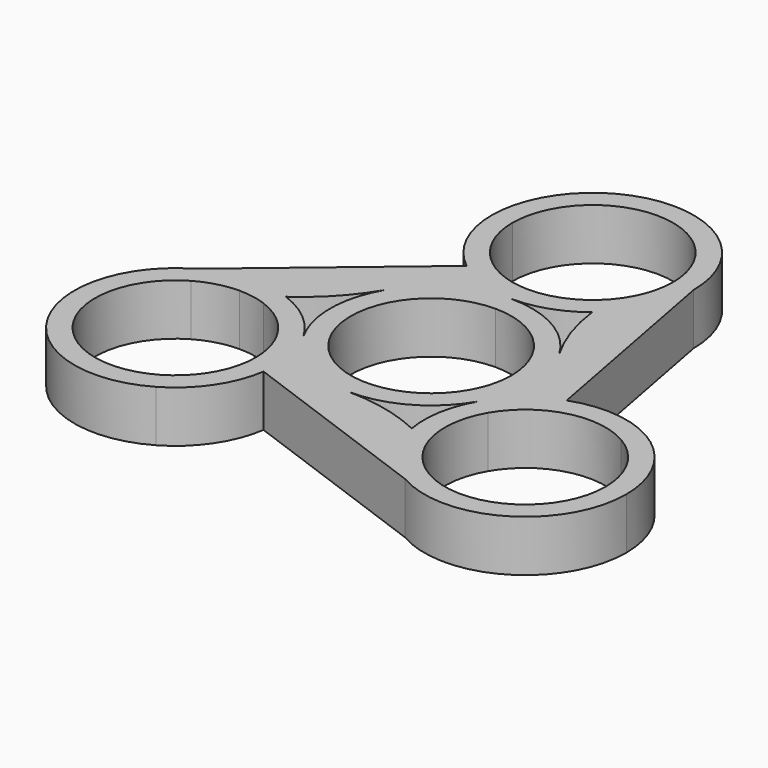
from build123d import *

# Parameters (mm, degrees)
F1_DEPTH = 7.112


# Not quite as in the source:
# - ends of sketch curves that miss each other by under 0.0002 mm in the source are joined
# - a feature names something its author has since deleted; it is built from what else it names


with BuildPart() as f1:
    # F0 (on Top) → F1 (new body)
    with BuildSketch(Plane.XY):
        with BuildLine():
            ThreePointArc((0, 11.1125), (7.8577241059, 7.8577241059), (11.1125, 0))
            ThreePointArc((11.1125, 0), (10.7338507446, -2.8761266387), (9.6237072996, -5.55625))
            Line((9.6237072996, -5.55625), (12.0983748909, -6.985))
            ThreePointArc((12.0983748909, -6.985), (13.4939838315, -3.6157019175), (13.97, 0))
            ThreePointArc((13.97, 0), (13.4755323786, 3.6838739276), (12.0271328398, 7.1069666985))
            ThreePointArc((12.0271328398, 7.1069666985), (6.9237480813, 12.133532565), (-1.95e-08, 13.97))
            Line((-1.95e-08, 13.97), (0, 11.1125))
        make_face()
        with BuildLine():
            ThreePointArc((-9.6237072996, -5.55625), (-9.6237072996, 5.55625), (0, 11.1125))
            Line((0, 11.1125), (0, 13.97))
            ThreePointArc((-1.95e-08, 13.97), (-6.9237478038, 12.1335327234), (-12.0271324949, 7.1069672823))
            ThreePointArc((-12.0271324949, 7.1069672823), (-13.9698214779, 0.0706248839), (-12.0983748909, -6.985))
            Line((-12.0983748909, -6.985), (-9.6237072996, -5.55625))
        make_face()
        with BuildLine():
            Line((12.0983748909, -6.985), (9.6237072996, -5.55625))
            ThreePointArc((9.6237072996, -5.55625), (0, -11.1125), (-9.6237072996, -5.55625))
            Line((-9.6237072996, -5.55625), (-12.0983748909, -6.985))
            ThreePointArc((-12.0983748909, -6.985), (-7.0460734842, -12.0629079602), (-0.1412475033, -13.969285921))
            ThreePointArc((-0.1412475033, -13.969285921), (6.9237481232, -12.1335325411), (12.0983748909, -6.985))
        make_face()
        with BuildLine():
            ThreePointArc((-8.6769039474, 16.9913819188), (-4.593947408, 14.7469507993), (-1.95e-08, 13.97))
            Line((0, 13.97), (0, 16.8275))
            ThreePointArc((0, 16.8275), (-3.65427634, 17.4455290423), (-6.9020826854, 19.2308719809))
            Line((-6.9020826854, 19.2308719809), (-8.6769039474, 16.9913819188))
        make_face()
        with BuildLine():
            ThreePointArc((-12.0271324949, 7.1069672823), (-6.9237478038, 12.1335327234), (-1.95e-08, 13.97))
            ThreePointArc((-1.95e-08, 13.97), (-4.593947408, 14.7469507993), (-8.6769039474, 16.9913819188))
            ThreePointArc((-8.6769039474, 16.9913819188), (-9.8388621787, 11.8752452293), (-12.0271324949, 7.1069672823))
        make_face()
        with BuildLine():
            Line((0, 16.8275), (0, 13.97))
            ThreePointArc((-1.95e-08, 13.97), (4.5939473896, 14.7469507929), (8.6769039474, 16.9913819188))
            ThreePointArc((8.6769039474, 16.9913819188), (12.5773059147, 21.8595168015), (13.97, 27.94))
            Line((13.97, 27.94), (11.1125, 27.94))
            ThreePointArc((11.1125, 27.94), (7.8577241059, 20.0822758941), (0, 16.8275))
        make_face()
        with BuildLine():
            ThreePointArc((19.4187283795, -0.8424940876), (15.2170069875, -3.2683590347), (12.0983750385, -6.9849997443))
            Line((12.0983750385, -6.9849997443), (14.5730424822, -8.41375))
            ThreePointArc((14.5730424822, -8.41375), (21.320623143, -3.2361492554), (29.7529997817, -4.3462927004))
            Line((29.7529997817, -4.3462927004), (31.1817497817, -1.8716251091))
            ThreePointArc((31.1817497817, -1.8716251091), (25.4143155079, -0.0531600677), (19.4187283795, -0.8424940876))
        make_face()
        with BuildLine():
            ThreePointArc((13.97, 0), (13.4939838315, -3.6157019175), (12.0983750385, -6.9849997443))
            ThreePointArc((12.0983750385, -6.9849997443), (15.2170069875, -3.2683590347), (19.4187283795, -0.8424940876))
            ThreePointArc((19.4187283795, -0.8424940876), (15.2933094518, 2.7327644521), (12.0271328398, 7.1069666985))
            ThreePointArc((12.0271328398, 7.1069666985), (13.4755323786, 3.6838739276), (13.97, 0))
        make_face()
        with BuildLine():
            Line((14.5730424822, -8.41375), (12.0983748909, -6.985))
            ThreePointArc((12.0983748909, -6.985), (10.4389854978, -11.5441348126), (10.4389854722, -16.395865042))
            ThreePointArc((10.4389854722, -16.395865042), (12.753195723, -21.9828628158), (17.2117497817, -26.0683748909))
            Line((17.2117497817, -26.0683748909), (18.6404997817, -23.5937072996))
            ThreePointArc((18.6404997817, -23.5937072996), (13.4628990371, -16.8461266387), (14.5730424822, -8.41375))
        make_face()
        with BuildLine():
            ThreePointArc((-10.2267497817, -13.97), (-10.7027659885, -10.3542979399), (-12.0983748909, -6.985))
            Line((-12.0983748909, -6.985), (-14.5730424822, -8.41375))
            ThreePointArc((-14.5730424822, -8.41375), (-13.4628990371, -11.0938733613), (-13.0842497817, -13.97))
            ThreePointArc((-13.0842497817, -13.97), (-14.5730424822, -19.52625), (-18.6404997817, -23.5937072996))
            Line((-18.6404997817, -23.5937072996), (-17.2117497817, -26.0683748909))
            ThreePointArc((-17.2117497817, -26.0683748909), (-12.6422439072, -21.8220248341), (-10.3765164134, -16.010110204))
            ThreePointArc((-10.3765164134, -16.010110204), (-10.2642417492, -14.9928000402), (-10.2267497817, -13.97))
        make_face()
        with BuildLine():
            ThreePointArc((-0.1412475033, -13.969285921), (-7.0460734842, -12.0629079602), (-12.0983748909, -6.985))
            ThreePointArc((-12.0983748909, -6.985), (-10.7027659885, -10.3542979399), (-10.2267497817, -13.97))
            ThreePointArc((-10.2267497817, -13.97), (-10.2642417492, -14.9928000402), (-10.3765164134, -16.010110204))
            ThreePointArc((-10.3765164134, -16.010110204), (-5.36483273, -14.4583271608), (-0.1412475033, -13.969285921))
        make_face()
        with BuildLine():
            Line((-14.5730424822, -8.41375), (-12.0983748909, -6.985))
            ThreePointArc((-12.0983748909, -6.985), (-15.2170068744, -3.2683591296), (-19.4187283795, -0.8424940876))
            Line((-19.4187283795, -0.8424940876), (-20.396050939, -3.5276657515))
            ThreePointArc((-20.396050939, -3.5276657515), (-17.0537724691, -5.4573311258), (-14.5730424822, -8.41375))
        make_face()
        with BuildLine():
            ThreePointArc((8.6769039474, 16.9913819188), (9.8388622875, 11.8752449082), (12.0271328398, 7.1069666985))
            ThreePointArc((12.0271328398, 7.1069666985), (15.2933094518, 2.7327644521), (19.4187283795, -0.8424940876))
            Line((19.4187283795, -0.8424940876), (13.97, 27.94))
            ThreePointArc((13.97, 27.94), (12.5773059147, 21.8595168015), (8.6769039474, 16.9913819188))
        make_face()
        with BuildLine():
            ThreePointArc((-19.4187283795, -0.8424940876), (-15.293309221, 2.7327647003), (-12.0271324949, 7.1069672823))
            ThreePointArc((-12.0271324949, 7.1069672823), (-9.8388621787, 11.8752452293), (-8.6769039474, 16.9913819188))
            Line((-8.6769039474, 16.9913819188), (-31.1817497817, -1.8716251091))
            ThreePointArc((-31.1817497817, -1.8716251091), (-27.8124518418, -0.4760162067), (-24.1967497817, 0))
            ThreePointArc((-24.1967497817, 0), (-21.7708847397, -0.2122356904), (-19.4187283795, -0.8424940876))
        make_face()
        with BuildLine():
            ThreePointArc((-13.97, 27.94), (-12.5773059147, 21.8595168015), (-8.6769039474, 16.9913819188))
            Line((-8.6769039474, 16.9913819188), (-6.9020826854, 19.2308719809))
            ThreePointArc((-6.9020826854, 19.2308719809), (-10.0046751594, 23.1032520012), (-11.1125, 27.94))
            Line((-11.1125, 27.94), (-13.97, 27.94))
        make_face()
        with BuildLine():
            ThreePointArc((10.4389854722, -16.395865042), (5.2800111814, -14.6107766948), (-0.1412475033, -13.969285921))
            ThreePointArc((-0.1412475033, -13.969285921), (-5.36483273, -14.4583271608), (-10.3765164134, -16.010110204))
            Line((-10.3765164134, -16.010110204), (17.2117497817, -26.0683748909))
            ThreePointArc((17.2117497817, -26.0683748909), (12.753195723, -21.9828628158), (10.4389854722, -16.395865042))
        make_face()
        with BuildLine():
            Line((-20.396050939, -3.5276657515), (-19.4187283795, -0.8424940876))
            ThreePointArc((-19.4187283795, -0.8424940876), (-21.7708847397, -0.2122356904), (-24.1967497817, 0))
            Line((-24.1967497817, 0), (-24.1967497817, -2.8575))
            ThreePointArc((-24.1967497817, -2.8575), (-22.2670844074, -3.0263238447), (-20.396050939, -3.5276657515))
        make_face()
        with BuildLine():
            ThreePointArc((-11.1125, 27.94), (0, 39.0525), (11.1125, 27.94))
            Line((11.1125, 27.94), (13.97, 27.94))
            ThreePointArc((13.97, 27.94), (0, 41.91), (-13.97, 27.94))
            Line((-13.97, 27.94), (-11.1125, 27.94))
        make_face()
        with BuildLine():
            Line((-29.7529997817, -4.3462927004), (-31.1817497817, -1.8716251091))
            ThreePointArc((-31.1817497817, -1.8716251091), (-36.2951246726, -20.955), (-17.2117497817, -26.0683748909))
            Line((-17.2117497817, -26.0683748909), (-18.6404997817, -23.5937072996))
            ThreePointArc((-18.6404997817, -23.5937072996), (-33.8204570813, -19.52625), (-29.7529997817, -4.3462927004))
        make_face()
        with BuildLine():
            ThreePointArc((-24.1967497817, 0), (-27.8124518418, -0.4760162067), (-31.1817497817, -1.8716251091))
            Line((-31.1817497817, -1.8716251091), (-29.7529997817, -4.3462927004))
            ThreePointArc((-29.7529997817, -4.3462927004), (-27.0728764204, -3.2361492554), (-24.1967497817, -2.8575))
            Line((-24.1967497817, -2.8575), (-24.1967497817, 0))
        make_face()
        with BuildLine():
            Line((31.1817497817, -1.8716251091), (29.7529997817, -4.3462927004))
            ThreePointArc((29.7529997817, -4.3462927004), (33.8204570813, -8.41375), (35.3092497817, -13.97))
            ThreePointArc((35.3092497817, -13.97), (29.7529997817, -23.5937072996), (18.6404997817, -23.5937072996))
            Line((18.6404997817, -23.5937072996), (17.2117497817, -26.0683748909))
            ThreePointArc((17.2117497817, -26.0683748909), (31.1817497817, -26.0683748909), (38.1667497817, -13.97))
            ThreePointArc((38.1667497817, -13.97), (36.2951246726, -6.985), (31.1817497817, -1.8716251091))
        make_face()
    extrude(amount=F1_DEPTH)


solid = f1.part
